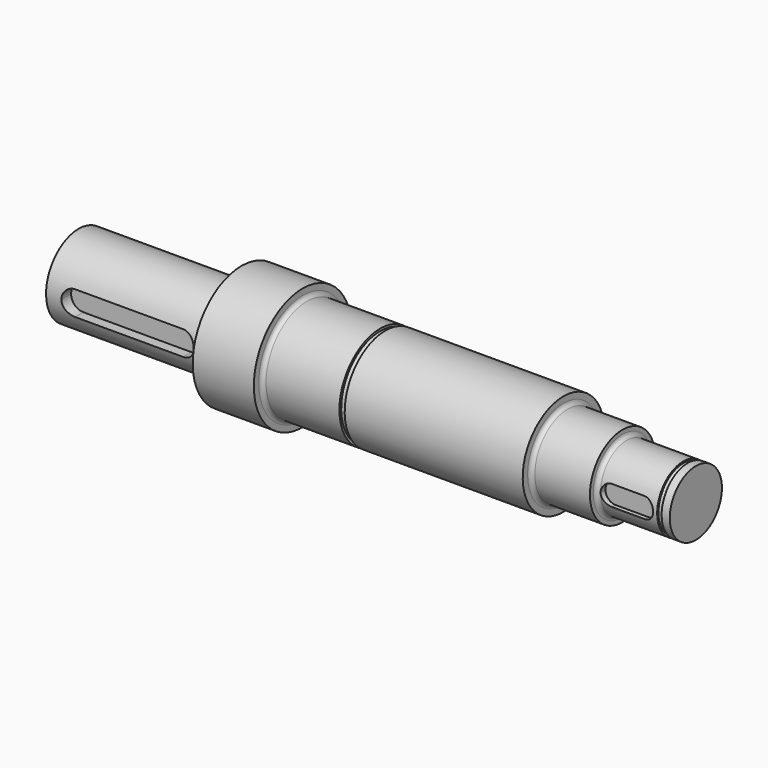
from build123d import *

# Parameters (mm, degrees)
F4_DEPTH = 3.5
F5_DEPTH = 3
F6_R     = 0.99999


# Not quite as in the source:
# - a fillet or chamfer is up to 0.001 mm smaller than in the source, because OpenCascade refuses the exact size


with BuildPart() as f1:
    # F0 (on Front) → F1 (revolve)
    with BuildSketch(Plane.XZ):
        Polygon((-75.75, 10), (-75.75, 0), (75.75, 0), (75.75, 8), (73.75, 8), (73.75, 7.6), (72.65, 7.6), (72.65, 8), (57.75, 8), (57.75, 10), (43.25, 10), (43.25, 12.5), (-0.45, 12.5), (-0.45, 11.95), (-1.75, 11.95), (-1.75, 12.5), (-20.75, 12.5), (-20.75, 15), (-35.75, 15), (-35.75, 10), align=None)
    revolve(axis=Axis((8.9792497456, 0, 0), (1, 0, 0)))

    # F3 (on offset) → F4 (cut)
    with BuildSketch(Plane.XZ.offset(10)):
        with BuildLine():
            Line((61.25, -2.5), (69.15, -2.5))
            ThreePointArc((69.15, -2.5), (70.917766953, -1.767766953), (71.65, 0))
            ThreePointArc((71.65, 0), (70.917766953, 1.767766953), (69.15, 2.5))
            Line((69.15, 2.5), (61.25, 2.5))
            ThreePointArc((61.25, 2.5), (59.482233047, 1.767766953), (58.75, 0))
            ThreePointArc((58.75, 0), (59.482233047, -1.767766953), (61.25, -2.5))
        make_face()
    extrude(amount=-F4_DEPTH, mode=Mode.SUBTRACT)

    # F3 (on offset) → F5 (cut)
    with BuildSketch(Plane.XZ.offset(10)):
        with BuildLine():
            Line((-69, -3), (-42.5, -3))
            ThreePointArc((-42.5, -3), (-40.3786796564, -2.1213203436), (-39.5, 0))
            ThreePointArc((-39.5, 0), (-40.3786796564, 2.1213203436), (-42.5, 3))
            Line((-42.5, 3), (-69, 3))
            ThreePointArc((-69, 3), (-71.1213203436, 2.1213203436), (-72, 0))
            ThreePointArc((-72, 0), (-71.1213203436, -2.1213203436), (-69, -3))
        make_face()
    extrude(amount=-F5_DEPTH, mode=Mode.SUBTRACT)

    # F6 (radius 1 in the source; OpenCascade refuses exactly that, so slightly less here)
    f6_edges = [f1.edges().sort_by_distance(p)[0] for p in [
        (-35.75, 0, -10),
        (-20.75, 0, -12.5),
        (43.25, 0, -10),
        (57.75, 0, -8),
    ]]
    fillet(f6_edges, radius=F6_R)


solid = f1.part
